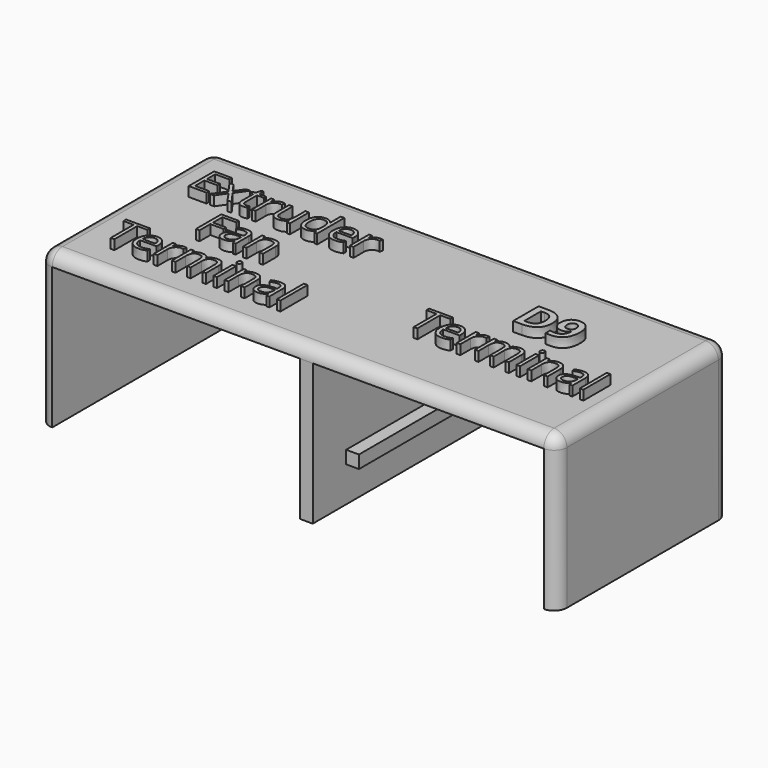
from build123d import *

# Parameters (mm, degrees)
F1_DEPTH     = 33.5
F2_W         = 18
F2_H         = 2
F3_DEPTH     = 2
F4_W         = 18
F4_H         = 2
F5_DEPTH     = 2
F6_TEXT_SIZE = 6.9444444444
F7_DEPTH     = 1.5
F8_W         = 2
F8_H         = 22
F9_DEPTH     = 3
F10_W        = 2
F10_H        = 22
F11_DEPTH    = 3
F12_W        = 3
F12_H        = 3.5
F13_DEPTH    = 2
F14_W        = 3
F14_H        = 3.5
F15_DEPTH    = 2
F16_R        = 1.99999


# Not quite as in the source:
# - a fillet or chamfer is up to 0.001 mm smaller than in the source, because OpenCascade refuses the exact size
# - Text() gives the source's letters only with a copy of the font that has no kerning and outlines rounded to 1/6400 em; it was checked with that copy


with BuildPart() as f1:
    # F0 (on Front) → F1 (new body)
    with BuildSketch(Plane.XZ):
        Polygon((-2, 0), (0, 0), (0, 24), (-80.6, 24), (-80.6, 0), (-78.6, 0), (-78.6, 22), (-40, 22), (-40, 0), (-38, 0), (-38, 22), (-2, 22), align=None)
    extrude(amount=-F1_DEPTH)

    # F2 (on face) → F3 (join)
    with BuildSketch(Plane.YZ.offset(-38)):
        with Locations((15.5, 6.5)):
            Rectangle(F2_W, F2_H)
    extrude(amount=F3_DEPTH)

    # F4 (on face) → F5 (join)
    with BuildSketch(Plane(origin=(-2, 0, 0), x_dir=(0, -1, 0), z_dir=(-1, 0, 0))):
        with Locations((-15.5, 6.5)):
            Rectangle(F4_W, F4_H)
    extrude(amount=F5_DEPTH)

    # F6 (on face) → F7 (join)
    with BuildSketch(Plane.XY.offset(24)):
        with Locations((-22.3574527155, 18.7003306186)):
            Text('D9', F6_TEXT_SIZE, font='Open Sans', font_style=FontStyle.BOLD, text_align=(TextAlign.LEFT, TextAlign.BOTTOM))
        with Locations((-31.8155235377, 9.8897580802)):
            Text('Terminal', F6_TEXT_SIZE, font='Open Sans', text_align=(TextAlign.LEFT, TextAlign.BOTTOM))
        with Locations((-75.4507258534, 21.7952029958)):
            Text('Extruder', F6_TEXT_SIZE, font='Open Sans', text_align=(TextAlign.LEFT, TextAlign.BOTTOM))
        with Locations((-67.70523265, 13.4952029958)):
            Text('Fan', F6_TEXT_SIZE, font='Open Sans', text_align=(TextAlign.LEFT, TextAlign.BOTTOM))
        with Locations((-75.2746909857, 5.1952029958)):
            Text('Terminal', F6_TEXT_SIZE, font='Open Sans', text_align=(TextAlign.LEFT, TextAlign.BOTTOM))
    extrude(amount=F7_DEPTH)

    # F8 (on face) → F9 (join)
    with BuildSketch(Plane(origin=(-2, 0, 0), x_dir=(0, -1, 0), z_dir=(-1, 0, 0))):
        with Locations((-32.5, 11)):
            Rectangle(F8_W, F8_H)
    extrude(amount=F9_DEPTH)

    # F10 (on face) → F11 (join)
    with BuildSketch(Plane.YZ.offset(-78.6)):
        with Locations((32.5, 11)):
            Rectangle(F10_W, F10_H)
    extrude(amount=F11_DEPTH)

    # F12 (on face) → F13 (cut, through all)
    with BuildSketch(Plane(origin=(0, 33.5, 0), x_dir=(-1, 0, 0), z_dir=(0, 1, 0))):
        with Locations((77.1, 1.75)):
            Rectangle(F12_W, F12_H)
    extrude(amount=-F13_DEPTH, mode=Mode.SUBTRACT)

    # F14 (on face) → F15 (cut, through all)
    with BuildSketch(Plane(origin=(0, 33.5, 0), x_dir=(-1, 0, 0), z_dir=(0, 1, 0))):
        with Locations((3.5, 1.75)):
            Rectangle(F14_W, F14_H)
    extrude(amount=-F15_DEPTH, mode=Mode.SUBTRACT)

    # F16 (radius 2 in the source; OpenCascade refuses exactly that, so slightly less here)
    f16_edges = [f1.edges().sort_by_distance(p)[0] for p in [
        (-80.6, 16.75, 24),
        (0, 16.75, 24),
        (0, 0, 12),
        (-40.3, 0, 24),
        (-80.6, 0, 12),
        (-40.3, 33.5, 24),
        (-80.6, 33.5, 12),
        (0, 33.5, 12),
    ]]
    fillet(f16_edges, radius=F16_R)


solid = f1.part
